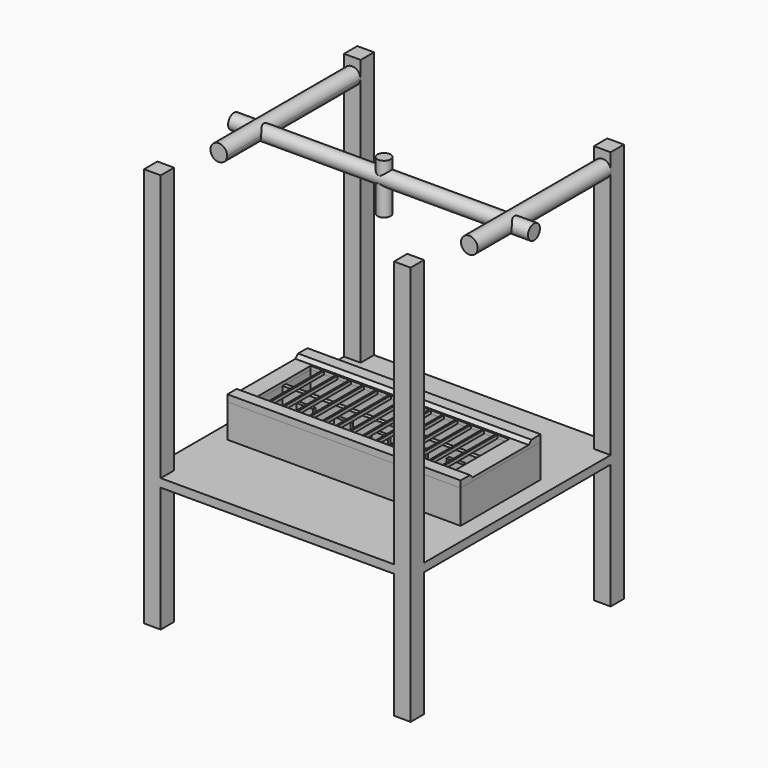
from build123d import *

# Parameters (mm, degrees)
F0_W           = 177.8
F0_H           = 76.2
F0_W_2         = 152.4
F0_H_2         = 23.8125
F1_DEPTH       = 25.4
F2_W           = 177.8
F2_H           = 76.2
F2_W_2         = 1.27
F2_H_2         = 23.8125
F2_H_3         = 3.175
F2_W_3         = 1.143
F3_DEPTH       = 2.54
F6_DEPTH       = 6.35
F4_W           = 177.8
F4_H           = 11.43
F7_DEPTH       = 2.54
F8_SIZE        = 2.53999
F5_W           = 12.7
F5_H           = 12.7
F9_DEPTH       = 101.6
F10_DEPTH      = 203.2
F11_R          = 6.35
F12_DEPTH      = 127
F14_DEPTH      = 203.2
F14_DEPTH_BACK = 25.4
F15_R          = 5.0551667009
F16_DEPTH      = 38.1
F17_W          = 12.7
F17_H          = 12.7
F19_DEPTH      = 2.54
F18_W          = 12.7
F18_H          = 12.7
F20_DEPTH      = 2.54


# Not quite as in the source:
# - a fillet or chamfer is up to 0.001 mm smaller than in the source, because OpenCascade refuses the exact size


with BuildPart() as f1:
    # F0 (on Top) → F1 (new body)
    with BuildSketch(Plane.XY):
        Rectangle(F0_W, F0_H)
        with Locations((0, -13.49375)):
            Rectangle(F0_W_2, F0_H_2, mode=Mode.SUBTRACT)
        with Locations((0, 13.49375)):
            Rectangle(F0_W_2, F0_H_2, mode=Mode.SUBTRACT)
    extrude(amount=F1_DEPTH)

    # F17 (on face) → F19 (join)
    with BuildSketch(Plane.XZ.offset(1.5875)):
        with Locations((57.15, 12.7)):
            Rectangle(F17_W, F17_H)
        with Locations((28.575, 12.7)):
            Rectangle(F17_W, F17_H)
        with Locations((0, 12.7)):
            Rectangle(F17_W, F17_H)
        with Locations((-28.575, 12.7)):
            Rectangle(F17_W, F17_H)
        with Locations((-57.15, 12.7)):
            Rectangle(F17_W, F17_H)
    extrude(amount=F19_DEPTH)

    # F18 (on face) → F20 (join)
    with BuildSketch(Plane(origin=(0, 1.5875, 0), x_dir=(-1, 0, 0), z_dir=(0, 1, 0))):
        with Locations((57.15, 12.7)):
            Rectangle(F18_W, F18_H)
        with Locations((28.575, 12.7)):
            Rectangle(F18_W, F18_H)
        with Locations((0, 12.7)):
            Rectangle(F18_W, F18_H)
        with Locations((-28.575, 12.7)):
            Rectangle(F18_W, F18_H)
        with Locations((-57.15, 12.7)):
            Rectangle(F18_W, F18_H)
    extrude(amount=F20_DEPTH)


with BuildPart() as f3:
    # F2 (on face) → F3 (new body)
    with BuildSketch(Plane.XY.offset(25.4)):
        Rectangle(F2_W, F2_H)
        Polygon((-76.2, 25.4), (-76.073, 25.4), (-67.183, 25.4), (-65.913, 25.4), (-57.023, 25.4), (-55.753, 25.4), (-46.863, 25.4), (-45.593, 25.4), (-36.703, 25.4), (-35.433, 25.4), (-26.543, 25.4), (-25.273, 25.4), (-16.383, 25.4), (-15.113, 25.4), (-6.223, 25.4), (-4.953, 25.4), (3.937, 25.4), (5.207, 25.4), (14.097, 25.4), (15.367, 25.4), (24.257, 25.4), (25.527, 25.4), (34.417, 25.4), (35.687, 25.4), (44.577, 25.4), (45.847, 25.4), (54.737, 25.4), (56.007, 25.4), (64.897, 25.4), (66.167, 25.4), (75.057, 25.4), (76.2, 25.4), (76.2, 1.5875), (75.057, 1.5875), (75.057, -1.5875), (76.2, -1.5875), (76.2, -25.4), (75.057, -25.4), (66.167, -25.4), (64.897, -25.4), (56.007, -25.4), (54.737, -25.4), (45.847, -25.4), (44.577, -25.4), (35.687, -25.4), (34.417, -25.4), (25.527, -25.4), (24.257, -25.4), (15.367, -25.4), (14.097, -25.4), (5.207, -25.4), (3.937, -25.4), (-4.953, -25.4), (-6.223, -25.4), (-15.113, -25.4), (-16.383, -25.4), (-25.273, -25.4), (-26.543, -25.4), (-35.433, -25.4), (-36.703, -25.4), (-45.593, -25.4), (-46.863, -25.4), (-55.753, -25.4), (-57.023, -25.4), (-65.913, -25.4), (-67.183, -25.4), (-76.073, -25.4), (-76.2, -25.4), (-76.2, -1.5875), (-76.073, -1.5875), (-76.073, 1.5875), (-76.2, 1.5875), align=None, mode=Mode.SUBTRACT)
        with Locations((-66.548, 13.49375)):
            Rectangle(F2_W_2, F2_H_2)
        with Locations((-66.548, 0)):
            Rectangle(F2_W_2, F2_H_3)
        with Locations((-66.548, -13.49375)):
            Rectangle(F2_W_2, F2_H_2)
        with Locations((-56.388, 13.49375)):
            Rectangle(F2_W_2, F2_H_2)
        with Locations((-56.388, 0)):
            Rectangle(F2_W_2, F2_H_3)
        with Locations((-56.388, -13.49375)):
            Rectangle(F2_W_2, F2_H_2)
        with Locations((-46.228, 13.49375)):
            Rectangle(F2_W_2, F2_H_2)
        with Locations((-46.228, 0)):
            Rectangle(F2_W_2, F2_H_3)
        with Locations((-46.228, -13.49375)):
            Rectangle(F2_W_2, F2_H_2)
        with Locations((-36.068, 13.49375)):
            Rectangle(F2_W_2, F2_H_2)
        with Locations((-36.068, 0)):
            Rectangle(F2_W_2, F2_H_3)
        with Locations((-36.068, -13.49375)):
            Rectangle(F2_W_2, F2_H_2)
        with Locations((-25.908, 13.49375)):
            Rectangle(F2_W_2, F2_H_2)
        with Locations((-25.908, 0)):
            Rectangle(F2_W_2, F2_H_3)
        with Locations((-25.908, -13.49375)):
            Rectangle(F2_W_2, F2_H_2)
        with Locations((-15.748, 13.49375)):
            Rectangle(F2_W_2, F2_H_2)
        with Locations((-15.748, 0)):
            Rectangle(F2_W_2, F2_H_3)
        with Locations((-15.748, -13.49375)):
            Rectangle(F2_W_2, F2_H_2)
        with Locations((-5.588, 13.49375)):
            Rectangle(F2_W_2, F2_H_2)
        with Locations((-5.588, 0)):
            Rectangle(F2_W_2, F2_H_3)
        with Locations((-5.588, -13.49375)):
            Rectangle(F2_W_2, F2_H_2)
        with Locations((4.572, 13.49375)):
            Rectangle(F2_W_2, F2_H_2)
        with Locations((4.572, 0)):
            Rectangle(F2_W_2, F2_H_3)
        with Locations((4.572, -13.49375)):
            Rectangle(F2_W_2, F2_H_2)
        with Locations((14.732, 13.49375)):
            Rectangle(F2_W_2, F2_H_2)
        with Locations((14.732, 0)):
            Rectangle(F2_W_2, F2_H_3)
        with Locations((14.732, -13.49375)):
            Rectangle(F2_W_2, F2_H_2)
        with Locations((24.892, 13.49375)):
            Rectangle(F2_W_2, F2_H_2)
        with Locations((24.892, 0)):
            Rectangle(F2_W_2, F2_H_3)
        with Locations((24.892, -13.49375)):
            Rectangle(F2_W_2, F2_H_2)
        with Locations((35.052, 13.49375)):
            Rectangle(F2_W_2, F2_H_2)
        with Locations((35.052, 0)):
            Rectangle(F2_W_2, F2_H_3)
        with Locations((35.052, -13.49375)):
            Rectangle(F2_W_2, F2_H_2)
        with Locations((75.6285, 13.49375)):
            Rectangle(F2_W_3, F2_H_2)
        with Locations((75.6285, -13.49375)):
            Rectangle(F2_W_3, F2_H_2)
        with Locations((65.532, 13.49375)):
            Rectangle(F2_W_2, F2_H_2)
        with Locations((65.532, 0)):
            Rectangle(F2_W_2, F2_H_3)
        with Locations((65.532, -13.49375)):
            Rectangle(F2_W_2, F2_H_2)
        with Locations((55.372, 13.49375)):
            Rectangle(F2_W_2, F2_H_2)
        with Locations((55.372, 0)):
            Rectangle(F2_W_2, F2_H_3)
        with Locations((55.372, -13.49375)):
            Rectangle(F2_W_2, F2_H_2)
        with Locations((45.212, 13.49375)):
            Rectangle(F2_W_2, F2_H_2)
        with Locations((45.212, 0)):
            Rectangle(F2_W_2, F2_H_3)
        with Locations((45.212, -13.49375)):
            Rectangle(F2_W_2, F2_H_2)
    extrude(amount=F3_DEPTH)

    # F4 (on face) → F7 (join)
    with BuildSketch(Plane.XY.offset(27.94)):
        with Locations((0, 32.385)):
            Rectangle(F4_W, F4_H)
        with Locations((0, -32.385)):
            Rectangle(F4_W, F4_H)
    extrude(amount=F7_DEPTH)

    # F8 (size 2.54 in the source; OpenCascade refuses exactly that, so slightly less here)
    f8_edges = [f3.edges().sort_by_distance(p)[0] for p in [
        (0, 26.67, 30.48),
        (0, -26.67, 30.48),
    ]]
    chamfer(f8_edges, length=F8_SIZE)


with BuildPart() as f6:
    # F5 (on Top) → F6 (new body)
    with BuildSketch(Plane.XY):
        Polygon((-88.9, -101.6), (88.9, -101.6), (88.9, -88.9), (101.6, -88.9), (101.6, 88.9), (88.9, 88.9), (88.9, 101.6), (-88.9, 101.6), (-88.9, 88.9), (-101.6, 88.9), (-101.6, -88.9), (-88.9, -88.9), align=None)
    extrude(amount=-F6_DEPTH)

    # F5 (on Top) → F9 (join)
    with BuildSketch(Plane.XY):
        with Locations((-95.25, 95.25)):
            Rectangle(F5_W, F5_H)
        with Locations((95.25, 95.25)):
            Rectangle(F5_W, F5_H)
        with Locations((95.25, -95.25)):
            Rectangle(F5_W, F5_H)
        with Locations((-95.25, -95.25)):
            Rectangle(F5_W, F5_H)
    extrude(amount=-F9_DEPTH)

    # F5 (on Top) → F10 (join)
    with BuildSketch(Plane.XY):
        with Locations((-95.25, 95.25)):
            Rectangle(F5_W, F5_H)
        with Locations((95.25, 95.25)):
            Rectangle(F5_W, F5_H)
        with Locations((95.25, -95.25)):
            Rectangle(F5_W, F5_H)
        with Locations((-95.25, -95.25)):
            Rectangle(F5_W, F5_H)
    extrude(amount=F10_DEPTH)

    # F11 (on face) → F12 (join)
    with BuildSketch(Plane.XZ.offset(-88.9)):
        with BuildLine():
            ThreePointArc((-101.6, 188.8838370386), (-94.6442935487, 184.2024947428), (-89.1091110349, 190.5))
            ThreePointArc((-89.1091110349, 190.5), (-94.6442935487, 196.7975052572), (-101.6, 192.1161629614))
            Line((-101.6, 192.1161629614), (-101.6, 188.8838370386))
        make_face()
        with Locations((95.4911112785, 190.5)):
            Circle(F11_R)
    extrude(amount=F12_DEPTH)

    # F13 (on face) → F14 (join, two sides)
    with BuildSketch(Plane.YZ.offset(-88.9)) as f14_sk:
        with BuildLine():
            ThreePointArc((5.6959577846, 190.0099871874), (-4.0276503748, 194.0376375623), (0, 184.3140294029))
            ThreePointArc((0, 184.3140294029), (4.0276503748, 185.9823368126), (5.6959577846, 190.0099871874))
        make_face()
    extrude(amount=F14_DEPTH)
    extrude(f14_sk.sketch, amount=-F14_DEPTH_BACK)

    # F15 (on face) → F16 (join)
    with BuildSketch(Plane.XY.offset(203.2)):
        Circle(F15_R)
    extrude(amount=-F16_DEPTH)


solid = Compound([f1.part, f3.part, f6.part])
